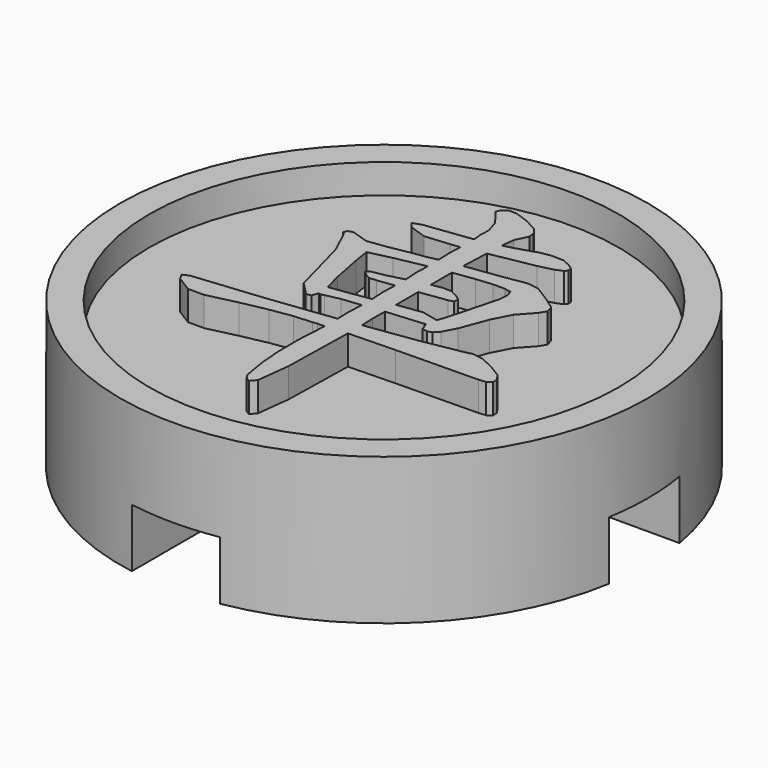
from build123d import *

# Parameters (mm, degrees)
F0_R     = 9
F1_DEPTH = 4
F3_W     = 3
F3_H     = 3
F4_DEPTH = 2
F2_R     = 9
F2_R_2   = 8
F5_DEPTH = 1
F7_DEPTH = 1


# Not quite as in the source:
# - a feature names something its author has since deleted; it is built from what else it names


with BuildPart() as f1:
    # F0 (on Top) → F1 (new body)
    with BuildSketch(Plane.XY):
        with Locations((-31.3306450844, 19.7580661625)):
            Circle(F0_R)
    extrude(amount=F1_DEPTH)

    # F3 (on face) → F4 (cut)
    with BuildSketch(Plane(origin=(0, 0, 0), x_dir=(1, 0, 0), z_dir=(0, 0, -1))):
        with BuildLine():
            ThreePointArc((-32.8306450844, -28.6321858371), (-32.0832814269, -28.7265408676), (-31.3306450844, -28.7580661625))
            ThreePointArc((-31.3306450844, -28.7580661625), (-30.5780087419, -28.7265408676), (-29.8306450844, -28.6321858371))
            Line((-29.8306450844, -28.6321858371), (-29.8306450844, -21.2580661625))
            Line((-29.8306450844, -21.2580661625), (-32.8306450844, -21.2580661625))
            Line((-32.8306450844, -21.2580661625), (-32.8306450844, -28.6321858371))
        make_face()
        with BuildLine():
            ThreePointArc((-40.204764759, -18.2580661625), (-40.2991197895, -19.0054298199), (-40.3306450844, -19.7580661625))
            ThreePointArc((-40.3306450844, -19.7580661625), (-40.2991197895, -20.510702505), (-40.204764759, -21.2580661625))
            Line((-40.204764759, -21.2580661625), (-32.8306450844, -21.2580661625))
            Line((-32.8306450844, -21.2580661625), (-32.8306450844, -18.2580661625))
            Line((-32.8306450844, -18.2580661625), (-40.204764759, -18.2580661625))
        make_face()
        with Locations((-31.3306450844, -19.7580661625)):
            Rectangle(F3_W, F3_H)
        with BuildLine():
            Line((-29.8306450844, -18.2580661625), (-29.8306450844, -21.2580661625))
            Line((-29.8306450844, -21.2580661625), (-22.4565254097, -21.2580661625))
            ThreePointArc((-22.4565254097, -21.2580661625), (-22.3621703793, -20.510702505), (-22.3306450844, -19.7580661625))
            ThreePointArc((-22.3306450844, -19.7580661625), (-22.3621703793, -19.0054298199), (-22.4565254097, -18.2580661625))
            Line((-22.4565254097, -18.2580661625), (-29.8306450844, -18.2580661625))
        make_face()
        with BuildLine():
            Line((-32.8306450844, -10.8839464878), (-32.8306450844, -18.2580661625))
            Line((-32.8306450844, -18.2580661625), (-29.8306450844, -18.2580661625))
            Line((-29.8306450844, -18.2580661625), (-29.8306450844, -10.8839464878))
            ThreePointArc((-29.8306450844, -10.8839464878), (-30.5780087419, -10.7895914574), (-31.3306450844, -10.7580661625))
            ThreePointArc((-31.3306450844, -10.7580661625), (-32.0832814269, -10.7895914574), (-32.8306450844, -10.8839464878))
        make_face()
    extrude(amount=-F4_DEPTH, mode=Mode.SUBTRACT)

    # F2 (on face) → F5 (join)
    with BuildSketch(Plane.XY.offset(4)):
        with Locations((-31.3306450844, 19.7580661625)):
            Circle(F2_R)
        with Locations((-31.3306450844, 19.7580661625)):
            Circle(F2_R_2, mode=Mode.SUBTRACT)
    extrude(amount=F5_DEPTH)

    # F6 (on face) → F7 (join)
    with BuildSketch(Plane.XY.offset(4)):
        Polygon((-31.8826989997, 17.620101061), (-31.6466835645, 17.6265811855), (-31.7066879875, 16.579484876), (-31.6994015259, 15.6946153355), (-31.6409921199, 14.9638444516), (-31.5461033208, 14.3823088935), (-31.5023139233, 14.1560195308), (-31.4098559066, 14.0027283885), (-31.2557513645, 13.9021557962), (-31.0951431551, 14.0935678455), (-30.9597079636, 15.2290645897), (-30.9069900022, 17.6882277109), (-29.3254158456, 17.7312048856), (-26.5207167102, 17.7758241628), (-26.2806401616, 17.8001378726), (-26.131438384, 17.902336676), (-26.1387366169, 18.0799662479), (-26.2968846155, 18.3046282224), (-26.7843359457, 18.5990530635), (-27.2012180722, 18.7815383146), (-27.5588903414, 18.842378503), (-27.8670641117, 18.7685604085), (-29.2313039551, 18.5276657515), (-30.9069900022, 18.2916503163), (-30.9264421472, 18.7580132848), (-30.9199620226, 19.2844101047), (-29.6028075528, 19.3979623688), (-29.6133429052, 19.3346972837), (-29.5768517406, 19.3103600312), (-29.5127567758, 19.1319241223), (-29.336775192, 19.0962275234), (-29.1826294501, 19.1457083654), (-29.0253054456, 19.3103600312), (-28.7941751179, 19.7483540621), (-28.4575735534, 20.6534526562), (-28.1363924487, 21.2779812803), (-27.6789580441, 21.7857381779), (-27.5499441205, 22.0039200278), (-27.6172762047, 22.239935463), (-27.9798335815, 22.5019067104), (-28.5711081605, 22.8758234335), (-28.9742178152, 22.9277350579), (-29.6644305355, 22.8142004508), (-30.9329399287, 22.6389840043), (-30.8940120961, 23.59281596), (-29.4016352941, 23.8685596792), (-28.9044726056, 23.9918645013), (-28.6586869554, 24.0956877501), (-28.5857046263, 24.1807945629), (-28.5970639727, 24.3098084866), (-28.7698084371, 24.4362915714), (-29.0609726161, 24.562833513), (-29.4551949066, 24.5750168534), (-29.829876767, 24.5109218886), (-30.3684157276, 24.3390014182), (-30.88103419, 24.1962150228), (-30.890769091, 24.1840316823), (-30.8680562839, 24.222170835), (-30.8137197628, 24.6561214094), (-30.6182036345, 25.065705303), (-30.6417463214, 25.2798260395), (-30.8064097585, 25.4907096565), (-31.2273471128, 25.7194268588), (-31.7245451154, 25.8929953172), (-31.9767755761, 25.897821568), (-32.162527375, 25.7696904951), (-32.222531798, 25.6293760818), (-32.1138587557, 25.4907096565), (-31.8267439188, 25.1127318199), (-31.6856113971, 24.6731310006), (-31.6985893032, 24.3657223677), (-31.672633491, 24.021057433), (-33.2688158848, 23.8198851742), (-33.5632230689, 23.7177099135), (-33.4083239611, 23.5311341206), (-32.8202865015, 23.3291967246), (-32.0003006059, 23.4046510358), (-31.672633491, 23.4435553257), (-31.6904729619, 22.9942431481), (-31.672633491, 22.5124420627), (-32.0514000076, 22.4338094888), (-32.363658434, 22.3891960973), (-33.186075112, 22.2423485884), (-33.8495492258, 22.1523566681), (-34.4399939251, 22.3405215924), (-34.6022089228, 22.288609968), (-34.648440874, 22.167777128), (-34.5535461892, 22.0614818971), (-34.1845028022, 21.2650328026), (-33.8235934136, 19.9267487714), (-33.6346044953, 19.2146413523), (-33.2071693594, 18.7815383146), (-33.1990530181, 18.7555883881), (-33.1682415268, 18.7685604085), (-33.0336126723, 18.7896605415), (-32.954109019, 19.0086487285), (-32.8770773478, 18.9867422584), (-32.7659499804, 19.0216266346), (-32.2825597636, 19.1213711129), (-31.6369427778, 19.1968077671), (-31.6612800303, 18.6485280198), (-31.6466835645, 18.1781157092), (-33.8868408417, 17.9031488987), (-36.2730075081, 17.6622718987), (-36.4798311888, 17.5673595569), (-36.3638475537, 17.360560596), (-35.8309782607, 17.0328699384), (-35.2802618454, 17.0328699384), (-34.2810337038, 17.2680790366), (-33.4042569619, 17.4465208312), (-32.654822613, 17.560885318), (-32.0392343242, 17.6006253733), align=None)
        Polygon((-31.6758764961, 21.5699694534), (-31.6466835645, 21.0817529858), (-32.1901017469, 20.936553465), (-32.6523977163, 20.8546249149), (-32.7691870998, 20.7483885407), (-32.6167011174, 20.6177854857), (-32.4601716785, 20.5391529118), (-32.2273933628, 20.5529253835), (-31.6466835645, 20.6307928201), (-31.6653293724, 20.1173856777), (-31.6369427778, 19.6380271461), (-32.3620398743, 19.524474882), (-32.9930603943, 19.4368960871), (-33.1552636207, 20.0500535935), (-33.3628983469, 21.1125350488), (-33.4472400224, 21.6591962363), (-32.6832268646, 21.8351778202), (-31.6596614706, 22.0387632043), align=None, mode=Mode.SUBTRACT)
        Polygon((-30.9329399287, 19.7743098743), (-30.9329399287, 20.718371615), (-30.0180416913, 20.8449135566), (-29.8485343463, 20.8919400735), (-29.829876767, 21.0460269586), (-30.0180416913, 21.1847522406), (-30.2775998133, 21.3088222), (-30.5720011117, 21.318592415), (-30.9329399287, 21.2569105756), (-30.9329399287, 22.1523566681), (-30.2143288425, 22.2545319288), (-29.6530711891, 22.3080915413), (-29.2556706359, 22.3120937981), (-29.0253054456, 22.2626541558), (-28.9636824629, 22.070428118), (-28.9864011556, 21.7370636729), (-29.1802163247, 21.0022375611), (-29.328652965, 20.4287965674), (-29.4438355602, 20.0159755543), (-29.537888594, 19.7613025399), (-30.1016182294, 19.8886684755), align=None, mode=Mode.SUBTRACT)
    extrude(amount=F7_DEPTH)


solid = f1.part
